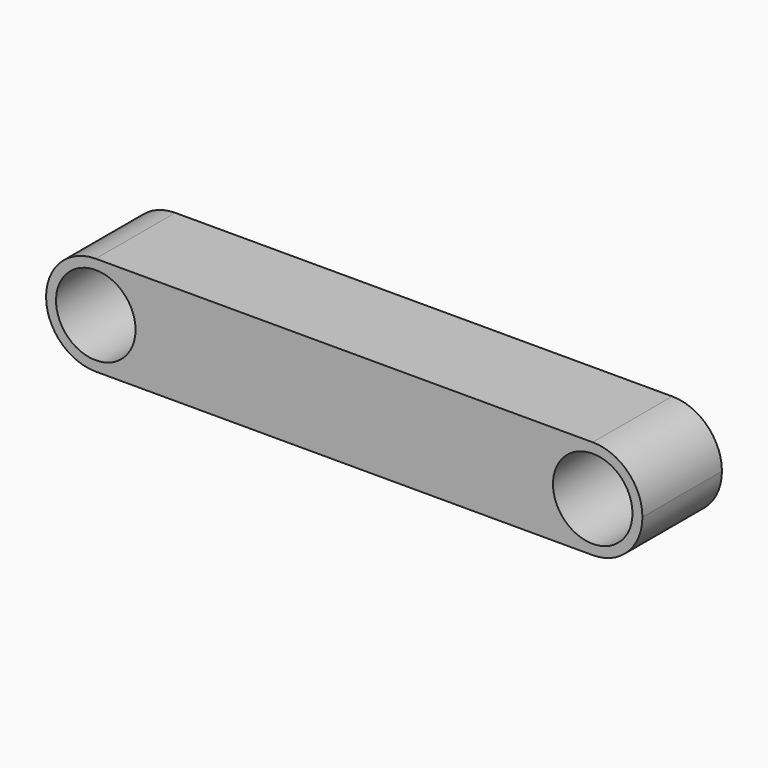
from build123d import *

# Parameters (mm, degrees)
F0_W     = 60
F0_H     = 10
F1_DEPTH = 10
F2_R     = 4
F3_DEPTH = 10.001
F4_R     = 4.99999
F5_R     = 4
F6_DEPTH = 10.001


# Not quite as in the source:
# - a fillet or chamfer is up to 0.001 mm smaller than in the source, because OpenCascade refuses the exact size


with BuildPart() as f1:
    # F0 (on Top) → F1 (new body)
    with BuildSketch(Plane.XY):
        Rectangle(F0_W, F0_H)
    extrude(amount=F1_DEPTH)

    # F2 (on face) → F3 (cut, through all)
    with BuildSketch(Plane.XZ.offset(5)):
        with Locations((-25, 5)):
            Circle(F2_R)
        with Locations((25, 5)):
            Circle(F2_R)
    extrude(amount=-F3_DEPTH, mode=Mode.SUBTRACT)

    # F4 (radius 5 in the source; OpenCascade refuses exactly that, so slightly less here)
    f4_edges = [f1.edges().sort_by_distance(p)[0] for p in [
        (-30, 0, 10),
        (-30, 0, 0),
        (30, 0, 10),
        (30, 0, 0),
    ]]
    fillet(f4_edges, radius=F4_R)

    # F5 (on face) → F6 (cut, through all)
    with BuildSketch(Plane.XZ.offset(5)):
        with Locations((45, 5)):
            Circle(F5_R)
    extrude(amount=-F6_DEPTH, mode=Mode.SUBTRACT)


solid = f1.part
